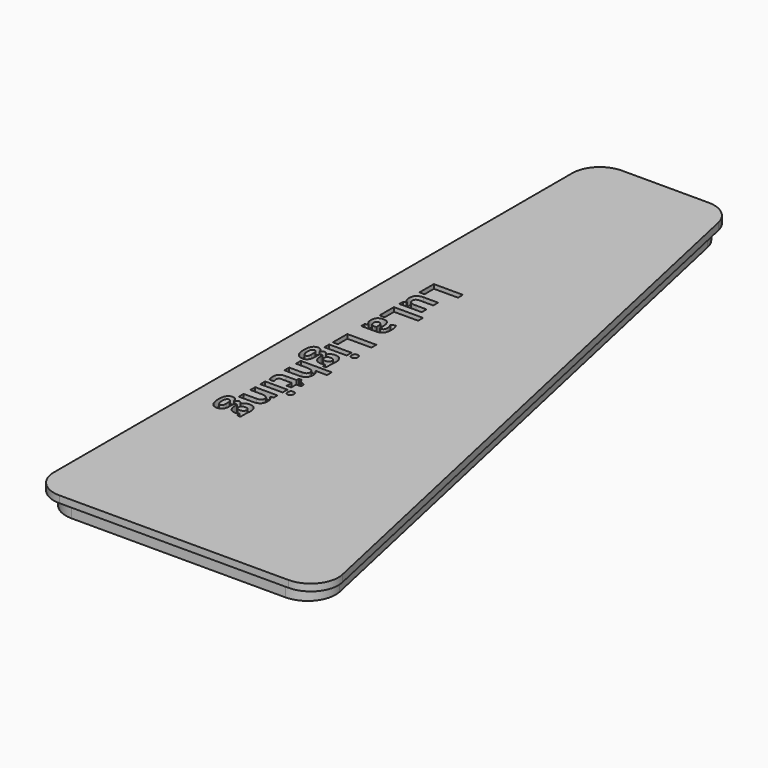
from build123d import *

# Parameters (mm, degrees)
F1_DEPTH     = 1
F2_DEPTH     = 3
F3_TEXT_SIZE = 5.9189382904
F4_DEPTH     = 25


# Not quite as in the source:
# - Text() gives the source's letters only with a copy of the font that has no kerning and outlines rounded to 1/6400 em; it was checked with that copy


with BuildPart() as f1:
    # F0 (on Top) → F1 (new body)
    with BuildSketch(Plane.XY):
        with BuildLine():
            ThreePointArc((3, 80.8347459125), (0.1715728753, 79.6631730373), (-1, 76.8347459125))
            Line((-1, 76.8347459125), (-1, -17.1652540875))
            ThreePointArc((-1, -17.1652540875), (0.1715728753, -19.9936812122), (3, -21.1652540875))
            Line((3, -21.1652540875), (36.2682578233, -21.1652540875))
            ThreePointArc((36.2682578233, -21.1652540875), (39.385771939, -19.6714675138), (40.1748356901, -16.3058069568))
            Line((40.1748356901, -16.3058069568), (19.4948356901, 77.6941930432))
            ThreePointArc((19.4948356901, 77.6941930432), (18.0944712497, 79.9522600282), (15.5882578233, 80.8347459125))
            Line((15.5882578233, 80.8347459125), (3, 80.8347459125))
        make_face()
        with BuildLine():
            ThreePointArc((-0.05, 75.8347459125), (1.1362175362, 78.6985283763), (4, 79.8847459125))
            Line((4, 79.8847459125), (14.7843437644, 79.8847459125))
            ThreePointArc((14.7843437644, 79.8847459125), (17.3218848586, 78.9912289547), (18.7397538546, 76.7049361324))
            Line((18.7397538546, 76.7049361324), (38.9797538546, -15.2950638676))
            ThreePointArc((38.9797538546, -15.2950638676), (38.1808268065, -18.7027951817), (35.0243437644, -20.2152540875))
            Line((35.0243437644, -20.2152540875), (4, -20.2152540875))
            ThreePointArc((4, -20.2152540875), (1.1362175362, -19.0290365513), (-0.05, -16.1652540875))
            Line((-0.05, -16.1652540875), (-0.05, 75.8347459125))
        make_face(mode=Mode.SUBTRACT)
    extrude(amount=-F1_DEPTH)



with BuildPart() as f1b:
    # F0 (on Top) → F1, piece 2 (new body)
    with BuildSketch(Plane.XY):
        with BuildLine():
            Line((14.7843437644, 78.8347459125), (4, 78.8347459125))
            ThreePointArc((4, 78.8347459125), (1.8786796564, 77.9560662561), (1, 75.8347459125))
            Line((1, 75.8347459125), (1, -16.1652540875))
            ThreePointArc((1, -16.1652540875), (1.8786796564, -18.286574431), (4, -19.1652540875))
            Line((4, -19.1652540875), (35.0243437644, -19.1652540875))
            ThreePointArc((35.0243437644, -19.1652540875), (37.3624793512, -18.0449141572), (37.9542771645, -15.5206687394))
            Line((37.9542771645, -15.5206687394), (17.7142771645, 76.4793312606))
            ThreePointArc((17.7142771645, 76.4793312606), (16.6640038342, 78.1728814993), (14.7843437644, 78.8347459125))
        make_face()
    extrude(amount=-F1_DEPTH)


with BuildPart() as f1_1:
    add(f1.part)

    add(f1b.part)  # F2 merges F1b
    # F0 (on Top) → F2 (join)
    with BuildSketch(Plane.XY):
        with BuildLine():
            Line((14.7843437644, 79.8847459125), (4, 79.8847459125))
            ThreePointArc((4, 79.8847459125), (1.1362175362, 78.6985283763), (-0.05, 75.8347459125))
            Line((-0.05, 75.8347459125), (-0.05, -16.1652540875))
            ThreePointArc((-0.05, -16.1652540875), (1.1362175362, -19.0290365513), (4, -20.2152540875))
            Line((4, -20.2152540875), (35.0243437644, -20.2152540875))
            ThreePointArc((35.0243437644, -20.2152540875), (38.1808268065, -18.7027951817), (38.9797538546, -15.2950638676))
            Line((38.9797538546, -15.2950638676), (18.7397538546, 76.7049361324))
            ThreePointArc((18.7397538546, 76.7049361324), (17.3218848586, 78.9912289547), (14.7843437644, 79.8847459125))
        make_face()
        with BuildLine():
            Line((0, -16.1652540875), (0, 75.8347459125))
            ThreePointArc((0, 75.8347459125), (1.1715728753, 78.6631730373), (4, 79.8347459125))
            Line((4, 79.8347459125), (14.7843437644, 79.8347459125))
            ThreePointArc((14.7843437644, 79.8347459125), (17.2905571908, 78.9522600282), (18.6909216312, 76.6941930432))
            Line((18.6909216312, 76.6941930432), (38.9309216312, -15.3058069568))
            ThreePointArc((38.9309216312, -15.3058069568), (38.1418578801, -18.6714675138), (35.0243437644, -20.1652540875))
            Line((35.0243437644, -20.1652540875), (4, -20.1652540875))
            ThreePointArc((4, -20.1652540875), (1.1715728753, -18.9936812122), (0, -16.1652540875))
        make_face(mode=Mode.SUBTRACT)
        with BuildLine():
            ThreePointArc((4, 79.8347459125), (1.1715728753, 78.6631730373), (0, 75.8347459125))
            Line((0, 75.8347459125), (0, -16.1652540875))
            ThreePointArc((0, -16.1652540875), (1.1715728753, -18.9936812122), (4, -20.1652540875))
            Line((4, -20.1652540875), (35.0243437644, -20.1652540875))
            ThreePointArc((35.0243437644, -20.1652540875), (38.1418578801, -18.6714675138), (38.9309216312, -15.3058069568))
            Line((38.9309216312, -15.3058069568), (18.6909216312, 76.6941930432))
            ThreePointArc((18.6909216312, 76.6941930432), (17.2905571908, 78.9522600282), (14.7843437644, 79.8347459125))
            Line((14.7843437644, 79.8347459125), (4, 79.8347459125))
        make_face()
        with BuildLine():
            ThreePointArc((1, 75.8347459125), (1.8786796564, 77.9560662561), (4, 78.8347459125))
            Line((4, 78.8347459125), (14.7843437644, 78.8347459125))
            ThreePointArc((14.7843437644, 78.8347459125), (16.6640038342, 78.1728814993), (17.7142771645, 76.4793312606))
            Line((17.7142771645, 76.4793312606), (37.9542771645, -15.5206687394))
            ThreePointArc((37.9542771645, -15.5206687394), (37.3624793512, -18.0449141572), (35.0243437644, -19.1652540875))
            Line((35.0243437644, -19.1652540875), (4, -19.1652540875))
            ThreePointArc((4, -19.1652540875), (1.8786796564, -18.286574431), (1, -16.1652540875))
            Line((1, -16.1652540875), (1, 75.8347459125))
        make_face(mode=Mode.SUBTRACT)
    extrude(amount=-F2_DEPTH)

    # F3 (on face) → F4 (cut)
    with BuildSketch(Plane.XY):
        with Locations(Location((3.7533092623, 46.3249027982), (0, 0, -90))):
            Text('LuLa Lighting', F3_TEXT_SIZE, font='Open Sans', font_style=FontStyle.BOLD, text_align=(TextAlign.LEFT, TextAlign.BOTTOM))
    extrude(amount=-F4_DEPTH, mode=Mode.SUBTRACT)


solid = f1_1.part
